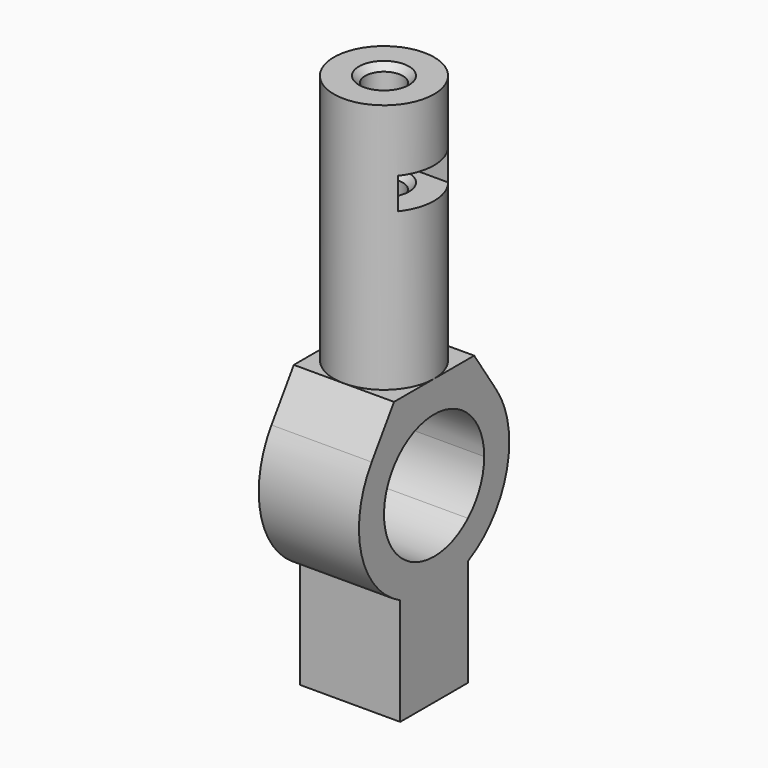
from build123d import *

# Parameters (mm, degrees)
F0_R     = 8
F0_R_2   = 3
F1_DEPTH = 40
F3_DEPTH = 8
F4_W     = 10
F4_H     = 5
F5_DEPTH = 8.001
F7_DEPTH = 5
F8_SIZE  = 1


with BuildPart() as f1:
    # F0 (on Top) → F1 (new body)
    with BuildSketch(Plane.XY):
        Circle(F0_R)
        Circle(F0_R_2, mode=Mode.SUBTRACT)
    extrude(amount=F1_DEPTH)

    # F2 (on Right) → F3 (join, symmetric)
    with BuildSketch(Plane.YZ):
        with BuildLine():
            ThreePointArc((6.762197, -28.389275), (12.77562, -22.86025), (15, -15))
            ThreePointArc((15, -15), (14.350108, -10.632576), (12.456747, -6.643599))
            ThreePointArc((12.456747, -6.643599), (7.058824, -1.764706), (0, 0))
            ThreePointArc((0, 0), (-7.058824, -1.764706), (-12.456747, -6.643599))
            ThreePointArc((-12.456747, -6.643599), (-14.510705, -18.799925), (-6.762197, -28.389275))
            Line((-6.762197, -28.389275), (-6.762197, -22.367))
            ThreePointArc((-6.762197, -22.367), (-4.023558, -5.845166), (10, -15))
            ThreePointArc((10, -15), (9.154834, -19.023558), (6.762197, -22.367))
            Line((6.762197, -22.367), (6.762197, -28.389275))
        make_face()
        with BuildLine():
            ThreePointArc((0, 0), (7.058824, -1.764706), (12.456747, -6.643599))
            Line((12.456747, -6.643599), (8, 0))
            Line((8, 0), (0, 0))
        make_face()
        with BuildLine():
            Line((6.762197, -45.492943), (6.762197, -28.389275))
            ThreePointArc((6.762197, -28.389275), (0, -30), (-6.762197, -28.389275))
            Line((-6.762197, -28.389275), (-6.762197, -45.492943))
            Line((-6.762197, -45.492943), (6.762197, -45.492943))
        make_face()
        with BuildLine():
            ThreePointArc((-6.762197, -28.389275), (0, -30), (6.762197, -28.389275))
            Line((6.762197, -28.389275), (6.762197, -22.367))
            ThreePointArc((6.762197, -22.367), (0, -25), (-6.762197, -22.367))
            Line((-6.762197, -22.367), (-6.762197, -28.389275))
        make_face()
        with BuildLine():
            ThreePointArc((-12.456747, -6.643599), (-7.058824, -1.764706), (0, 0))
            Line((0, 0), (-8, 0))
            Line((-8, 0), (-12.456747, -6.643599))
        make_face()
    extrude(amount=F3_DEPTH, both=True)

    # F4 (on Right) → F5 (cut, through all)
    with BuildSketch(Plane.YZ):
        with Locations((0, 27.5)):
            Rectangle(F4_W, F4_H)
    extrude(amount=F5_DEPTH, mode=Mode.SUBTRACT)

    # F6 (on face) → F7 (cut, through all)
    with BuildSketch(Plane(origin=(0, 0, 30), x_dir=(1, 0, 0), z_dir=(0, 0, -1))):
        Polygon((-2.886751, -5), (2.886751, -5), (5.773503, 0), (2.886751, 5), (-2.886751, 5), (-5.773503, 0), align=None)
    extrude(amount=F7_DEPTH, mode=Mode.SUBTRACT)

    # F8
    f8_edges = [f1.edges().sort_by_distance(p)[0] for p in [
        (-3, 0, 40),
        (-3, 0, 25),
    ]]
    chamfer(f8_edges, length=F8_SIZE)


solid = f1.part
